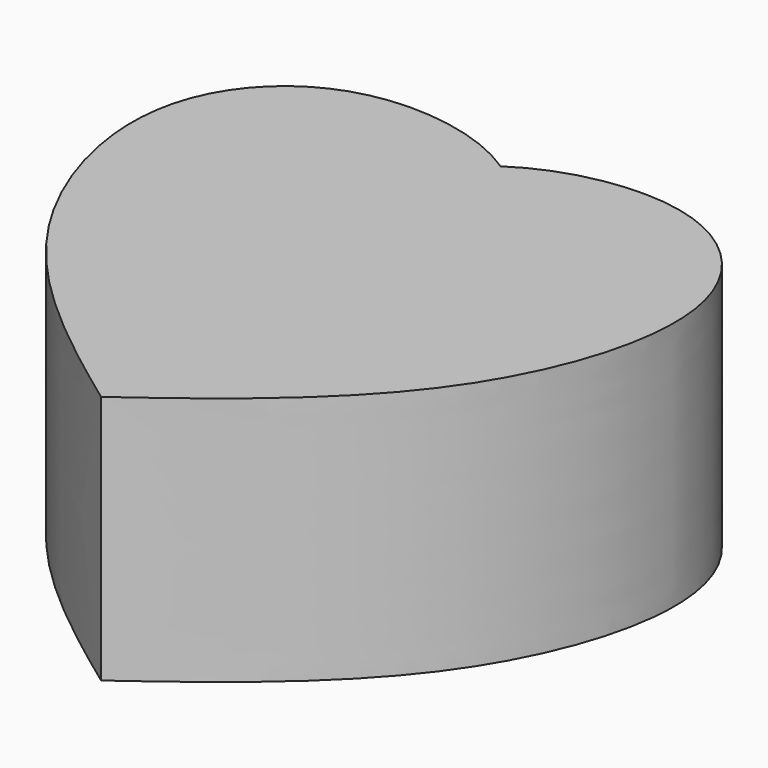
from build123d import *

# Parameters (mm, degrees)
F1_DEPTH = 12.7


# Not quite as in the source:
# - the dataset's text gives a spline's control points without its knots; the knots are read off the source's solid


with BuildPart() as f1:
    # F0 (on Top) → F1 (new body)
    with BuildSketch(Plane.XY):
        with BuildLine():
            add(Edge.make_bspline(
                [(0, 7.3985277553), (0.0561317913, 7.4355978201), (0.2884330841, 7.5858529945), (0.6234033364, 7.7839671378), (1.0097634379, 7.9872043524), (1.4099097954, 8.1805425071), (1.9266069091, 8.3981604537), (2.568217098, 8.6207931494), (3.2287477023, 8.8047516143), (4.1303838823, 8.9971318489), (5.289014144, 9.1349974082), (6.7048507265, 9.1183901501), (7.7665502497, 8.9486545011), (8.4635672947, 8.7578139959), (8.924916934, 8.608559512), (9.4854066891, 8.3824765368), (10.1275883188, 8.0490745126), (10.9366024292, 7.5233995043), (11.8465417819, 6.7180627841), (12.5860853692, 5.7314011473), (13.0561102842, 4.8482770761), (13.3438572483, 4.1436573712), (13.5269870465, 3.5249453278), (13.6379814755, 3.0138060633), (13.7247636765, 2.4981208728), (13.7905794586, 1.8444205109), (13.8124648138, 0.7838140306), (13.6961458361, -0.5644171318), (13.3556158381, -2.2032973109), (12.8335347256, -3.8468908713), (12.1444882554, -5.4759402949), (11.4408288043, -6.8032166551), (10.8051411167, -7.8352312055), (10.1220567014, -8.8426622927), (9.1946194769, -10.0397077732), (7.9822385799, -11.3908223198), (6.6887104132, -12.6672193119), (5.3304832165, -13.8808637723), (3.9231768508, -15.0430633389), (2.4817693359, -16.164685428), (1.1685813845, -17.1457503238), (0.3398869399, -17.7531588062), (0, -18.0014722447)],
                knots=[0.1229070341, 0.1229070341, 0.1229070341, 0.1229070341, 0.1280843465, 0.1440948898, 0.1521001615, 0.1601054331, 0.1761159765, 0.1921265198, 0.2081370631, 0.2241476064, 0.256168693, 0.2881897797, 0.3202108663, 0.3282161379, 0.3362214096, 0.3522319529, 0.3682424962, 0.3842530395, 0.4162741262, 0.4482952128, 0.4643057561, 0.4803162994, 0.4963268427, 0.5043321144, 0.5123373861, 0.5283479294, 0.5443584727, 0.5763795593, 0.6084006459, 0.6404217326, 0.6724428192, 0.7044639058, 0.7204744491, 0.7364849925, 0.7685060791, 0.8005271657, 0.8325482523, 0.864569339, 0.8965904256, 0.9286115122, 0.9606325989, 0.9829524144, 0.9829524144, 0.9829524144, 0.9829524144], degree=3))
            add(Edge.make_bspline(
                [(0, 7.3985277553), (-0.0561317913, 7.4355978201), (-0.2884330841, 7.5858529945), (-0.6234033364, 7.7839671378), (-1.0097634379, 7.9872043524), (-1.4099097954, 8.1805425071), (-1.9266069091, 8.3981604537), (-2.568217098, 8.6207931494), (-3.2287477023, 8.8047516143), (-4.1303838823, 8.9971318489), (-5.289014144, 9.1349974082), (-6.7048507265, 9.1183901501), (-7.7665502497, 8.9486545011), (-8.4635672947, 8.7578139959), (-8.924916934, 8.608559512), (-9.485406689, 8.3824765368), (-10.1275883188, 8.0490745126), (-10.9366024292, 7.5233995043), (-11.8465417818, 6.7180627841), (-12.5860853692, 5.7314011473), (-13.0561102842, 4.8482770761), (-13.3438572483, 4.1436573712), (-13.5269870465, 3.5249453278), (-13.6379814755, 3.0138060633), (-13.7247636764, 2.4981208728), (-13.7905794586, 1.8444205109), (-13.8124648138, 0.7838140306), (-13.6961458361, -0.5644171318), (-13.3556158381, -2.2032973109), (-12.8335347256, -3.8468908713), (-12.1444882554, -5.4759402949), (-11.4408288043, -6.8032166551), (-10.8051411167, -7.8352312055), (-10.1220567014, -8.8426622927), (-9.1946194769, -10.0397077732), (-7.9822385799, -11.3908223198), (-6.6887104132, -12.6672193119), (-5.3304832165, -13.8808637723), (-3.9231768508, -15.0430633389), (-2.4817693359, -16.164685428), (-1.1685813845, -17.1457503238), (-0.3398869399, -17.7531588062), (0, -18.0014722447)],
                knots=[0.1229070341, 0.1229070341, 0.1229070341, 0.1229070341, 0.1280843465, 0.1440948898, 0.1521001615, 0.1601054331, 0.1761159765, 0.1921265198, 0.2081370631, 0.2241476064, 0.256168693, 0.2881897797, 0.3202108663, 0.3282161379, 0.3362214096, 0.3522319529, 0.3682424962, 0.3842530395, 0.4162741262, 0.4482952128, 0.4643057561, 0.4803162994, 0.4963268427, 0.5043321144, 0.5123373861, 0.5283479294, 0.5443584727, 0.5763795593, 0.6084006459, 0.6404217326, 0.6724428192, 0.7044639058, 0.7204744491, 0.7364849925, 0.7685060791, 0.8005271657, 0.8325482523, 0.864569339, 0.8965904256, 0.9286115122, 0.9606325989, 0.9829524144, 0.9829524144, 0.9829524144, 0.9829524144], degree=3))
        make_face()
    extrude(amount=F1_DEPTH)


solid = f1.part
